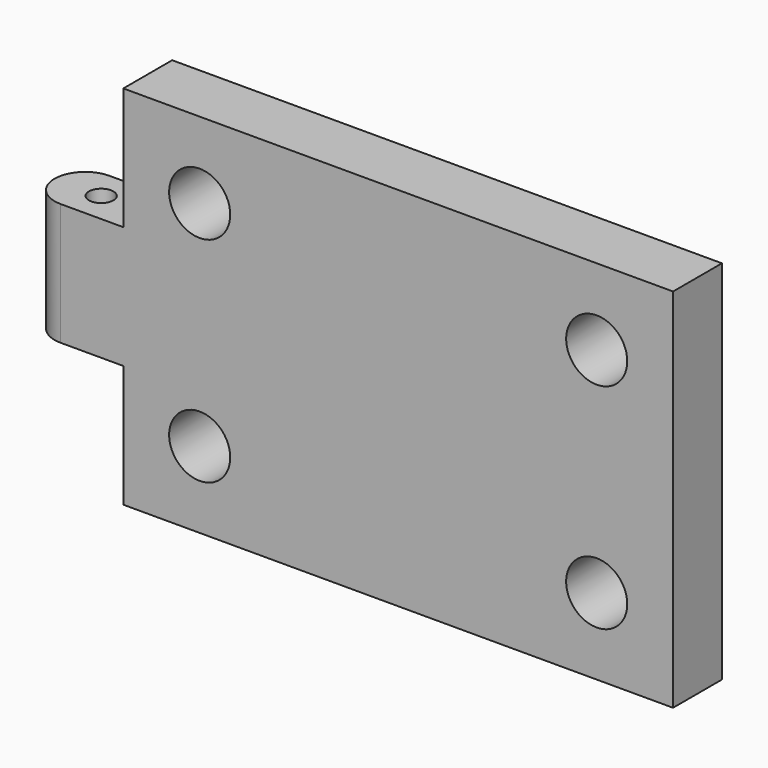
from build123d import *

# Parameters (mm, degrees)
F0_W     = 3.05
F0_H     = 4
F1_DEPTH = 2
F2_R     = 0.4
F3_DEPTH = 25
F4_R     = 1
F5_DEPTH = 25
F6_R     = 0.99999


# Not quite as in the source:
# - a fillet or chamfer is up to 0.001 mm smaller than in the source, because OpenCascade refuses the exact size


with BuildPart() as f1:
    # F0 (on Front) → F1 (new body)
    with BuildSketch(Plane.XZ):
        Polygon((9, -6), (9, 6), (-9, 6), (-9, 2), (-5.95, 2), (-5.95, -2), (-9, -2), (-9, -6), align=None)
        with Locations((-7.475, 0)):
            Rectangle(F0_W, F0_H)
        with Locations((-10.525, 0)):
            Rectangle(F0_W, F0_H)
    extrude(amount=F1_DEPTH)

    # F2 (on face) → F3 (cut)
    with BuildSketch(Plane(origin=(0, 0, -2), x_dir=(1, 0, 0), z_dir=(0, 0, -1))):
        with Locations((-10.525, 1)):
            Circle(F2_R)
    extrude(amount=-F3_DEPTH, mode=Mode.SUBTRACT)

    # F4 (on face) → F5 (cut)
    with BuildSketch(Plane.XZ.offset(2)):
        with Locations((-6.5, 3.5)):
            Circle(F4_R)
        with Locations((6.5, 3.5)):
            Circle(F4_R)
        with Locations((6.5, -3.5)):
            Circle(F4_R)
        with Locations((-6.5, -3.5)):
            Circle(F4_R)
    extrude(amount=-F5_DEPTH, mode=Mode.SUBTRACT)

    # F6 (radius 1 in the source; OpenCascade refuses exactly that, so slightly less here)
    f6_edges = [f1.edges().sort_by_distance(p)[0] for p in [
        (-12.05, -2, 0),
        (-12.05, 0, 0),
    ]]
    fillet(f6_edges, radius=F6_R)


solid = f1.part
